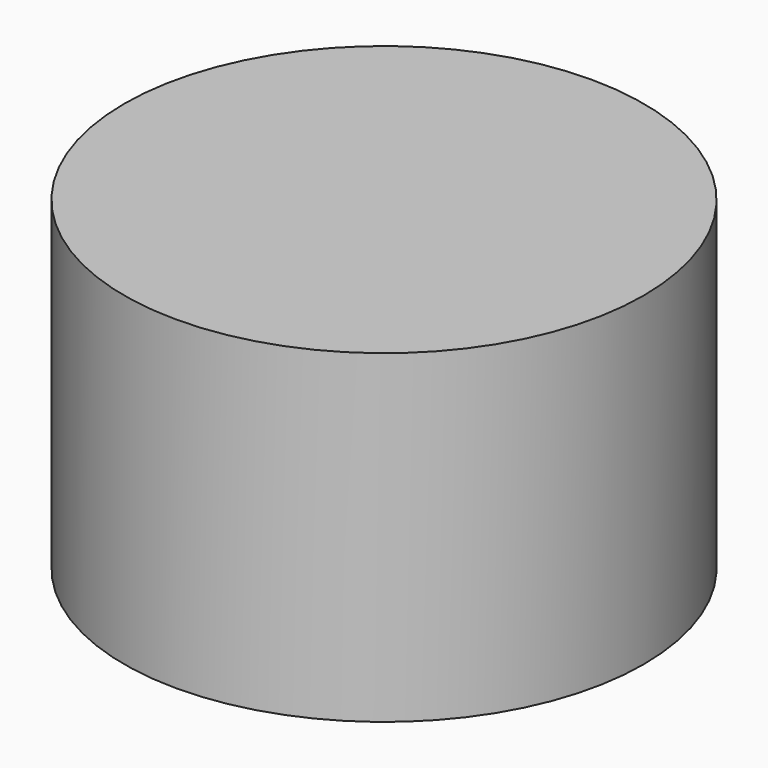
from build123d import *

# Parameters (mm, degrees)
F0_R     = 17.2
F1_DEPTH = 21.5
F2_T     = -0.025


# Not quite as in the source:
# - a feature names something its author has since deleted; it is built from what else it names


with BuildPart() as f1:
    # F0 (on Top) → F1 (new body)
    with BuildSketch(Plane.XY):
        Circle(F0_R)
    extrude(amount=-F1_DEPTH)

    # F2
    f2_openings = [f1.faces().sort_by_distance(p)[0] for p in [
        (0, 0, -21.5),
    ]]
    offset(amount=F2_T, openings=f2_openings)


solid = f1.part
